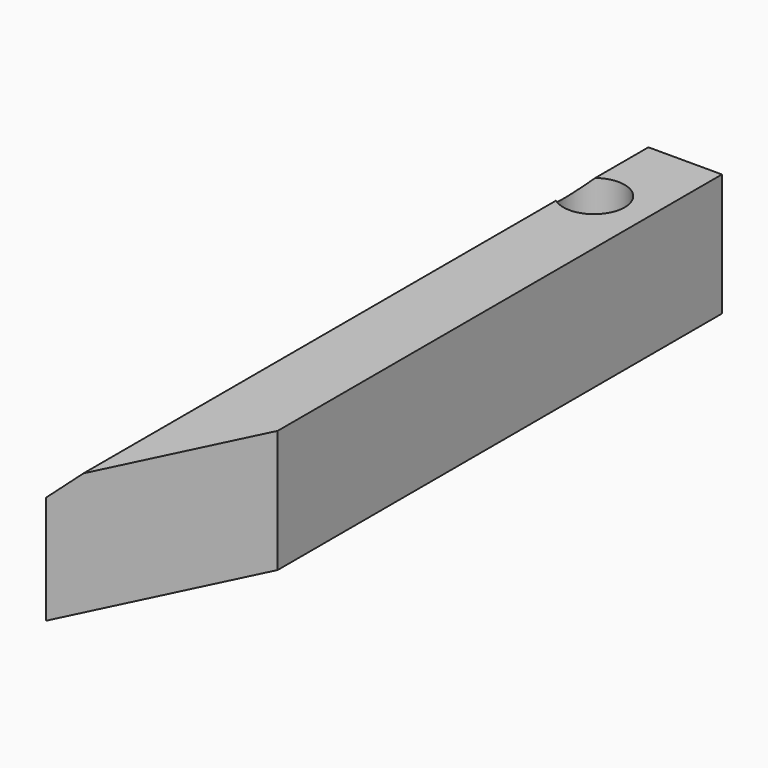
from build123d import *

# Parameters (mm, degrees)
F1_DEPTH = 12.7
F2_SIZE  = 12.69999
F4_D     = 6.35


# Not quite as in the source:
# - a fillet or chamfer is up to 0.001 mm smaller than in the source, because OpenCascade refuses the exact size


with BuildPart() as f1:
    # F0 (on Top) → F1 (new body)
    with BuildSketch(Plane.XY):
        Polygon((9.0852697523, 24.0329056978), (-11.2347302477, 24.0329056978), (-11.2347302477, 0), (-11.2347302477, -37.6667892456), (0, -52.1670943022), (9.0852697523, -33.5160031522), align=None)
    extrude(amount=F1_DEPTH)

    # F2 (size 12.7 in the source; OpenCascade refuses exactly that, so slightly less here)
    f2_edges = [f1.edges().sort_by_distance(p)[0] for p in [
        (-11.23473, -6.816942, 12.7),
    ]]
    chamfer(f2_edges, length=F2_SIZE)

    # F4 (through all)
    with Locations(Plane.XY.offset(12.7)):
        with Locations((3.3710829448, 14.6072776988)):
            Hole(F4_D / 2)


solid = f1.part
